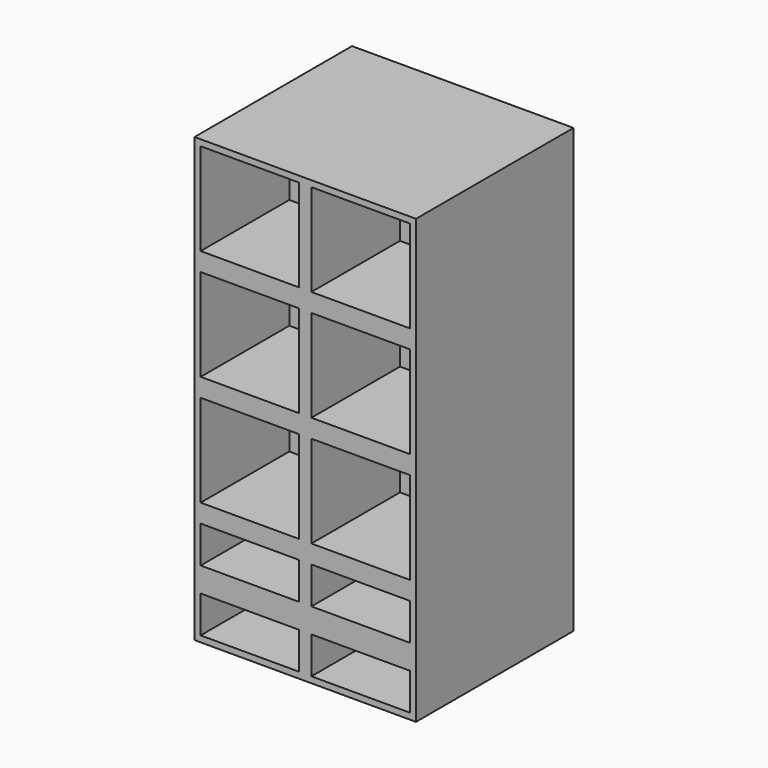
from build123d import *

# Parameters (mm, degrees)
F0_W     = 457.2
F0_H     = 1828.8
F1_DEPTH = 812.8
F2_W     = 406.4
F2_H     = 381
F2_H_2   = 152.4
F3_DEPTH = 457.2


with BuildPart() as f1:
    # F0 (on Front) → F1 (new body)
    with BuildSketch(Plane.XZ):
        with Locations((-228.6, 0)):
            Rectangle(F0_W, F0_H)
        with Locations((228.6, 0)):
            Rectangle(F0_W, F0_H)
    extrude(amount=-F1_DEPTH)

    # F2 (on face) → F3 (cut)
    with BuildSketch(Plane.XZ):
        with Locations((228.6, 698.5)):
            Rectangle(F2_W, F2_H)
        with Locations((228.6, 241.3)):
            Rectangle(F2_W, F2_H)
        with Locations((-228.6, 698.5)):
            Rectangle(F2_W, F2_H)
        with Locations((228.6, -215.9)):
            Rectangle(F2_W, F2_H)
        with Locations((-228.6, 241.3)):
            Rectangle(F2_W, F2_H)
        with Locations((228.6, -558.8)):
            Rectangle(F2_W, F2_H_2)
        with Locations((-228.6, -215.9)):
            Rectangle(F2_W, F2_H)
        with Locations((228.6, -812.8)):
            Rectangle(F2_W, F2_H_2)
        with Locations((-228.6, -558.8)):
            Rectangle(F2_W, F2_H_2)
        with Locations((-228.6, -812.8)):
            Rectangle(F2_W, F2_H_2)
    extrude(amount=-F3_DEPTH, mode=Mode.SUBTRACT)


solid = f1.part
